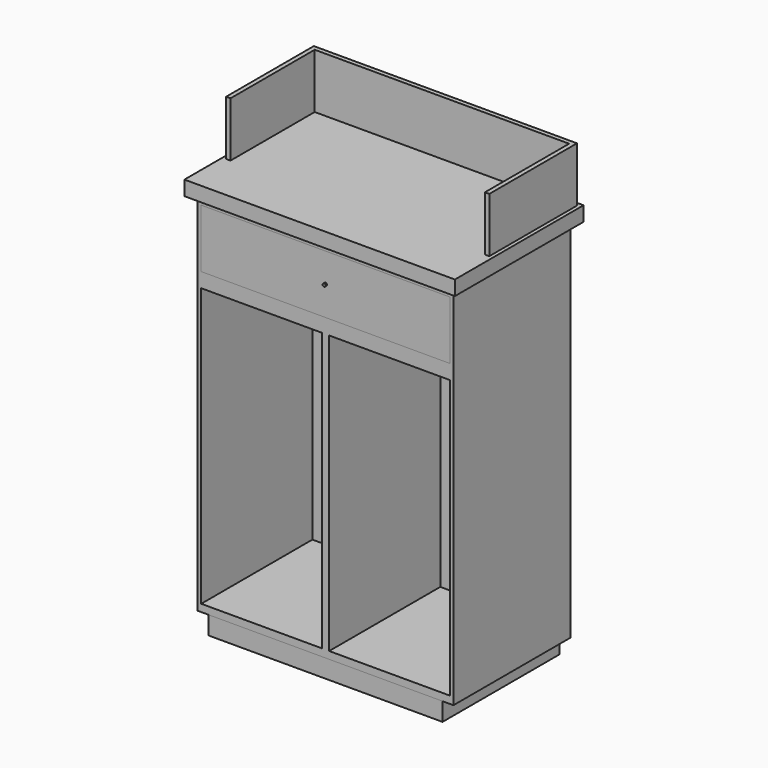
from build123d import *

# Parameters (mm, degrees)
F0_W          = 700
F0_H          = 400
F1_DEPTH      = 1000
F2_W          = 330
F2_H          = 760
F2_W_2        = 680
F2_H_2        = 160
F3_DEPTH      = 380
F4_W          = 680
F4_H          = 160
F5_DEPTH      = 10
F6_W          = 10
F6_H          = 160
F7_DEPTH      = 340
F8_W          = 680
F8_H          = 160
F9_DEPTH      = 20
F10_R         = 4
F11_DEPTH     = 5
F12_DEPTH     = 5
F13_W         = 740
F13_H         = 440
F14_DEPTH     = 40
F15_W         = 640
F15_H         = 399.7640275955
F16_DEPTH     = 50
F17_T         = 10
F17_T3_DEPTH  = 720
F17_T5_DEPTH  = 420
F17_T7_DEPTH  = 660
F17_T9_DEPTH  = 419.7640275955
F17_T11_DEPTH = 400
F17_T13_DEPTH = 700
F17_T15_DEPTH = 180
F17_T17_DEPTH = 350
F17_T19_DEPTH = 780
F17_T21_DEPTH = 350
F19_DEPTH     = 150


# Not quite as in the source:
# - a shell that OpenCascade refuses in one call is made with other operations: the cavity is built on its own and cut out


with BuildPart() as f1:
    # F0 (on Top) → F1 (new body)
    with BuildSketch(Plane.XY):
        Rectangle(F0_W, F0_H)
    extrude(amount=F1_DEPTH)

    # F2 (on face) → F3 (cut)
    with BuildSketch(Plane.XZ.offset(200)):
        with Locations((-175, 400)):
            Rectangle(F2_W, F2_H)
        with Locations((175, 400)):
            Rectangle(F2_W, F2_H)
        with Locations((0, 900)):
            Rectangle(F2_W_2, F2_H_2)
    extrude(amount=-F3_DEPTH, mode=Mode.SUBTRACT)

    # F13 (on face) → F14 (join)
    with BuildSketch(Plane.XY.offset(1000)):
        Rectangle(F13_W, F13_H)
    extrude(amount=F14_DEPTH)

    # F15 (on face) → F16 (join)
    with BuildSketch(Plane(origin=(0, 0, 0), x_dir=(1, 0, 0), z_dir=(0, 0, -1))):
        Rectangle(F15_W, F15_H)
    extrude(amount=F16_DEPTH)

    # F17: shell of thickness 10, made by hand


with BuildPart() as f5:
    # F4 (on face) → F5 (new body)
    with BuildSketch(Plane.XZ.offset(200)):
        with Locations((0, 900)):
            Rectangle(F4_W, F4_H)
    extrude(amount=-F5_DEPTH)


with BuildPart() as f7:
    # F6 (on face) → F7 (new body)
    with BuildSketch(Plane(origin=(0, -190, 0), x_dir=(-1, 0, 0), z_dir=(0, 1, 0))):
        with Locations((-335, 900)):
            Rectangle(F6_W, F6_H)
    extrude(amount=F7_DEPTH)


with BuildPart() as f7b:
    # F6 (on face) → F7, piece 2 (new body)
    with BuildSketch(Plane(origin=(0, -190, 0), x_dir=(-1, 0, 0), z_dir=(0, 1, 0))):
        with Locations((335, 900)):
            Rectangle(F6_W, F6_H)
    extrude(amount=F7_DEPTH)


with BuildPart() as f9:
    # F8 (on face) → F9 (new body)
    with BuildSketch(Plane(origin=(0, 150, 0), x_dir=(-1, 0, 0), z_dir=(0, 1, 0))):
        with Locations((0, 900)):
            Rectangle(F8_W, F8_H)
    extrude(amount=F9_DEPTH)


with BuildPart() as f11:
    # F10 (on face) → F11 (new body)
    with BuildSketch(Plane.XZ.offset(200)):
        with Locations((0, 900)):
            Circle(F10_R)
    extrude(amount=F11_DEPTH)


with BuildPart() as f12:
    # F10 (on face) → F12 (new body)
    with BuildSketch(Plane.XZ.offset(200)):
        with Locations((0, 900)):
            Circle(F10_R)
    extrude(amount=F12_DEPTH)


with BuildPart() as f17_core1:
    # F17_t2: copy of F1
    add(f1.part)

    # the walls: a layer under each face that stays
    f17_faces = [f17_core1.faces().sort_by_distance(p)[0] for p in [
        (0, -220, 1020),
        (-370, 0, 1020),
        (370, 0, 1020),
        (-345.3333333333, -205.3333333333, 1000),
        (0, 0, 1040),
        (0, 220, 1020),
        (0, -200, 500),
        (350, 0, 500),
        (0, 200, 500),
        (-350, 0, 500),
        (-326.6666666667, -186.6666666667, 0),
        (0, -10, 980),
        (340, -10, 900),
        (0, -10, 820),
        (-340, -10, 900),
        (-175, -10, 780),
        (-10, -10, 400),
        (-175, -10, 20),
        (-340, -10, 400),
        (175, -10, 20),
        (10, -10, 400),
        (175, -10, 780),
        (340, -10, 400),
        (0, -199.8820137978, -25),
        (320, 0, -25),
        (0, 199.8820137978, -25),
        (-320, 0, -25),
        (0, 180, 900),
        (-175, 180, 400),
        (175, 180, 400),
    ]]
    thicken(f17_faces, amount=-F17_T, mode=Mode.SUBTRACT)

    # F17_s4 → F17_t3 (cut)
    with BuildSketch(Plane.YZ.offset(-360)):
        Polygon((-200.1, 999.9), (-200, 1010), (-190, 1010), (-190, 1000), align=None)
        Polygon((200.1, 999.9), (200, 1010), (190, 1010), (190, 1000), align=None)
    extrude(amount=F17_T3_DEPTH, mode=Mode.SUBTRACT)

    # F17_s6 → F17_t5 (cut)
    with BuildSketch(Plane.XZ.offset(-210)):
        Polygon((350.1, 999.9), (350, 1010), (340, 1010), (340, 1000), align=None)
        Polygon((-350.1, 999.9), (-350, 1010), (-340, 1010), (-340, 1000), align=None)
    extrude(amount=F17_T5_DEPTH, mode=Mode.SUBTRACT)

    # F17_s8 → F17_t7 (cut)
    with BuildSketch(Plane.YZ.offset(-330)):
        Polygon((-199.9820137978, -0.1), (-199.8820137978, 10), (-189.8820137978, 10), (-189.8820137978, 0), align=None)
        Polygon((199.9820137978, -0.1), (199.8820137978, 10), (189.8820137978, 10), (189.8820137978, 0), align=None)
    extrude(amount=F17_T7_DEPTH, mode=Mode.SUBTRACT)

    # F17_s10 → F17_t9 (cut)
    with BuildSketch(Plane.XZ.offset(-209.8820137978)):
        Polygon((320.1, -0.1), (320, 10), (310, 10), (310, 0), align=None)
        Polygon((-320.1, -0.1), (-320, 10), (-310, 10), (-310, 0), align=None)
    extrude(amount=F17_T9_DEPTH, mode=Mode.SUBTRACT)

    # F17_s12 → F17_t11 (cut)
    with BuildSketch(Plane.XZ.offset(-190)):
        Polygon((339.9, 979.9), (340, 990), (350, 990), (350, 980), align=None)
        Polygon((-339.9, 979.9), (-340, 990), (-350, 990), (-350, 980), align=None)
        Polygon((339.9, 820.1), (350, 820), (350, 810), (340, 810), align=None)
        Polygon((-339.9, 820.1), (-340, 810), (-350, 810), (-350, 820), align=None)
        Polygon((-10.1, 779.9), (-10, 790), (0, 790), (0, 780), align=None)
        Polygon((-339.9, 779.9), (-340, 790), (-350, 790), (-350, 780), align=None)
        Polygon((-10.1, 20.1), (0, 20), (0, 10), (-10, 10), align=None)
        Polygon((-339.9, 20.1), (-340, 10), (-350, 10), (-350, 20), align=None)
        Polygon((10.1, 20.1), (10, 10), (0, 10), (0, 20), align=None)
        Polygon((339.9, 20.1), (340, 10), (350, 10), (350, 20), align=None)
        Polygon((10.1, 779.9), (0, 780), (0, 790), (10, 790), align=None)
        Polygon((339.9, 779.9), (340, 790), (350, 790), (350, 780), align=None)
    extrude(amount=F17_T11_DEPTH, mode=Mode.SUBTRACT)

    # F17_s14 → F17_t13 (cut)
    with BuildSketch(Plane.YZ.offset(-350)):
        Polygon((179.9, 979.9), (180, 990), (190, 990), (190, 980), align=None)
        Polygon((179.9, 820.1), (180, 810), (190, 810), (190, 820), align=None)
    extrude(amount=F17_T13_DEPTH, mode=Mode.SUBTRACT)

    # F17_s16 → F17_t15 (cut)
    with BuildSketch(Plane.XY.offset(810)):
        Polygon((339.9, 179.9), (350, 180), (350, 190), (340, 190), align=None)
        Polygon((-339.9, 179.9), (-350, 180), (-350, 190), (-340, 190), align=None)
    extrude(amount=F17_T15_DEPTH, mode=Mode.SUBTRACT)

    # F17_s18 → F17_t17 (cut)
    with BuildSketch(Plane.YZ.offset(-350)):
        Polygon((179.9, 779.9), (180, 790), (190, 790), (190, 780), align=None)
        Polygon((179.9, 20.1), (180, 10), (190, 10), (190, 20), align=None)
    extrude(amount=F17_T17_DEPTH, mode=Mode.SUBTRACT)

    # F17_s20 → F17_t19 (cut)
    with BuildSketch(Plane.XY.offset(10)):
        Polygon((-10.1, 179.9), (0, 180), (0, 190), (-10, 190), align=None)
        Polygon((-339.9, 179.9), (-350, 180), (-350, 190), (-340, 190), align=None)
        Polygon((10.1, 179.9), (0, 180), (0, 190), (10, 190), align=None)
        Polygon((339.9, 179.9), (350, 180), (350, 190), (340, 190), align=None)
    extrude(amount=F17_T19_DEPTH, mode=Mode.SUBTRACT)

    # F17_s22 → F17_t21 (cut)
    with BuildSketch(Plane.YZ):
        Polygon((179.9, 20.1), (180, 10), (190, 10), (190, 20), align=None)
        Polygon((179.9, 779.9), (180, 790), (190, 790), (190, 780), align=None)
    extrude(amount=F17_T21_DEPTH, mode=Mode.SUBTRACT)


with BuildPart() as f1_1:
    add(f1.part)

    # what is left inside the walls is the cavity
    f17_cavity = [f17_core1.part.solids().sort_by_distance(p)[0] for p in [
        (0, -70, 1029.9),
        (103.333333, 0, 9.9),
        (113.333333, 0, 809.9),
    ]]
    add(f17_cavity, mode=Mode.SUBTRACT)

    # F18 (on face) → F19 (join)
    with BuildSketch(Plane.XY.offset(1040)):
        Polygon((-348, 198), (348, 198), (348, -90), (360, -90), (360, 198), (360, 210), (348, 210), (-348, 210), (-360, 210), (-360, 198), (-360, -90), (-348, -90), align=None)
    extrude(amount=F19_DEPTH)


solid = Compound([f5.part, f7.part, f7b.part, f9.part, f11.part, f12.part, f1_1.part])
